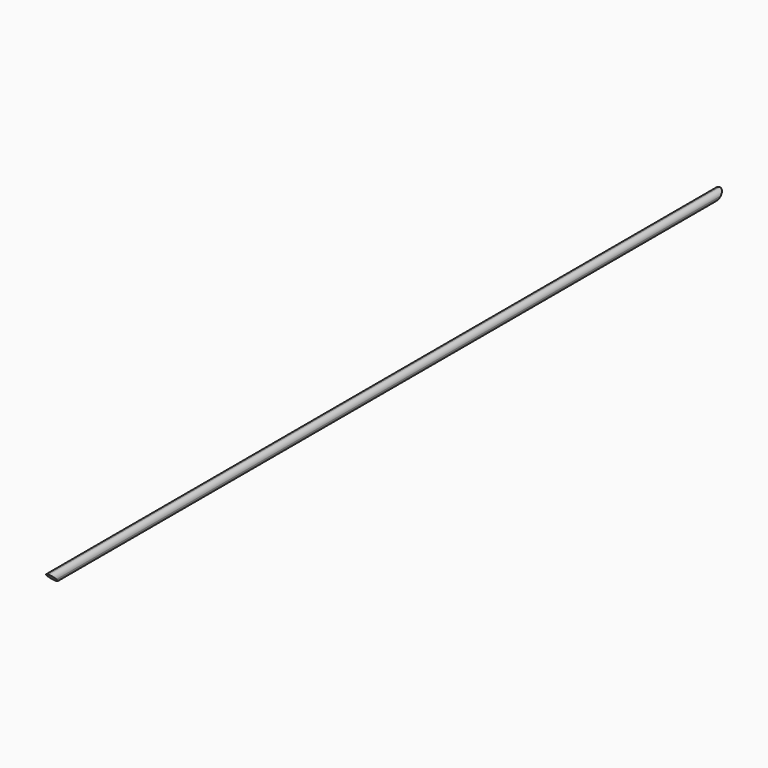
from build123d import *

# Parameters (mm, degrees)
F0_W     = 33
F0_H     = 33
F1_DEPTH = 1500
F3_DEPTH = 50
F4_R     = 16.49999


# Not quite as in the source:
# - a fillet or chamfer is up to 0.001 mm smaller than in the source, because OpenCascade refuses the exact size


with BuildPart() as f1:
    # F0 (on Front) → F1 (new body, symmetric)
    with BuildSketch(Plane.XZ):
        Rectangle(F0_W, F0_H)
    extrude(amount=F1_DEPTH, both=True)

    # F2 (on face) → F3 (cut)
    with BuildSketch(Plane.YZ.offset(16.5)):
        Polygon((1500, -16.5), (1500, 16.5), (1467, -16.5), align=None)
        Polygon((-1467, -16.5), (-1500, 16.5), (-1500, -16.5), align=None)
    extrude(amount=-F3_DEPTH, mode=Mode.SUBTRACT)

    # F4 (radius 16.5 in the source; OpenCascade refuses exactly that, so slightly less here)
    f4_edges = [f1.edges().sort_by_distance(p)[0] for p in [
        (16.5, 0, 16.5),
        (16.5, 0, -16.5),
        (-16.5, 0, -16.5),
        (-16.5, 0, 16.5),
    ]]
    fillet(f4_edges, radius=F4_R)


solid = f1.part
